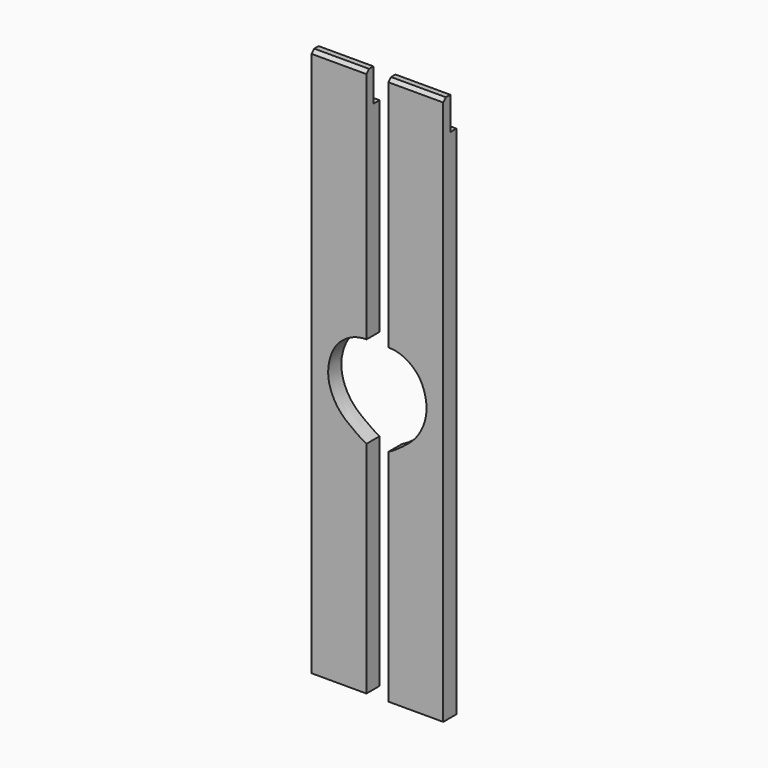
from build123d import *

# Parameters (mm, degrees)
F0_W     = 63.5
F0_H     = 635
F1_DEPTH = 19.05
F2_DEPTH = 19.05
F4_DEPTH = 25.4
F5_W     = 8.89
F5_H     = 38.1
F6_DEPTH = 203.2


# Not quite as in the source:
# - ends of sketch curves that miss each other by under 0.0002 mm in the source are joined
# - the dataset's text gives a spline's control points without its knots; the knots are read off the source's solid


with BuildPart() as f1:
    # F0 (on Front) → F1 (new body)
    with BuildSketch(Plane.XZ):
        with Locations((31.75, 317.5)):
            Rectangle(F0_W, F0_H)
    extrude(amount=F1_DEPTH)

    # F0 (on Front) → F2 (join)
    with BuildSketch(Plane.XZ):
        with Locations((31.75, 317.5)):
            Rectangle(F0_W, F0_H)
    extrude(amount=F2_DEPTH)


with BuildPart() as f2:
    # F0 (on Front) → F2, piece 2 (new body)
    with BuildSketch(Plane.XZ):
        with Locations((120.65, 317.5)):
            Rectangle(F0_W, F0_H)
    extrude(amount=F2_DEPTH)


with BuildPart() as f4_tool:
    # F3 (on Front) → F4 (new body)
    with BuildSketch(Plane.XZ):
        with BuildLine():
            add(Edge.make_bspline(
                [(76.100897188, 249.9055047823), (75.926185189, 249.9503102981), (75.0072900635, 250.1900406969), (73.2686411586, 250.6826857781), (70.8066541331, 251.4744223929), (68.2535936156, 252.4016337409), (66.0855662311, 253.2919660254), (64.3444467026, 254.0808435025), (62.6141081034, 254.9200047281), (60.530623259, 256.0298058039), (58.1240131579, 257.4465535403), (55.796019872, 258.9289142825), (53.5234926315, 260.4628622816), (51.6580388559, 261.7732381383), (50.1690572917, 262.8373998229), (49.0559378965, 263.6386485181), (47.9204267705, 264.459940904), (46.3757335395, 265.5883530434), (44.4005510811, 267.0614970435), (41.9904856802, 268.940615508), (39.5721301398, 270.9437516515), (37.1771637761, 273.0857076613), (35.2273267058, 275.0014654048), (33.7139364208, 276.6200965999), (32.6031412309, 277.8843862966), (31.5392969514, 279.1785289773), (30.1869925643, 280.9326379146), (28.6162502842, 283.1744606608), (26.9167867496, 285.9192166814), (25.3965198658, 288.697331361), (24.0503105367, 291.4878274589), (22.8732786897, 294.2731728334), (21.8629980956, 297.0286748974), (21.0083636149, 299.7731949442), (20.0799064427, 303.4278925622), (19.3201051185, 307.9921101901), (19.0525714688, 313.46912822), (19.3407698255, 318.0082202574), (19.8503150972, 321.6100699757), (20.3651164621, 324.2955196511), (20.8994087113, 326.5198480427), (21.3857760258, 328.2896704175), (21.9199810431, 330.0777026424), (22.6836120267, 332.3350954426), (23.7765594955, 335.0624054196), (25.0695252606, 337.7860696689), (26.5870492336, 340.482876144), (28.0551387249, 342.6818667185), (29.3671419532, 344.4023295399), (30.7492710306, 346.0639842696), (32.5901917449, 348.0257211027), (35.741037592, 350.9238010664), (39.1454385563, 353.4591937744), (42.7161593673, 355.6127823059), (45.4584424247, 357.0273277396), (48.2564247079, 358.2324558767), (51.1102551, 359.2200466799), (54.0138871108, 359.9816388995), (56.9592002347, 360.5106156141), (59.4398513134, 360.7540031429), (61.4342021839, 360.8300374212), (63.4344324402, 360.8265137523), (65.8869615803, 360.6817979446), (68.7271248443, 360.3158428641), (70.9786334936, 359.8645110662), (72.7038693594, 359.4132156878), (73.9618405888, 359.0249055159), (74.9862735439, 358.6517484591), (75.6947865713, 358.3571550213), (75.9996347623, 358.2212228776), (76.1008674062, 358.1750149305)],
                knots=[0.0119144147, 0.0119144147, 0.0119144147, 0.0119144147, 0.015625, 0.03125, 0.046875, 0.0625, 0.078125, 0.0859375, 0.09375, 0.109375, 0.125, 0.140625, 0.15625, 0.171875, 0.1796875, 0.1875, 0.1953125, 0.203125, 0.21875, 0.234375, 0.25, 0.265625, 0.28125, 0.2890625, 0.296875, 0.3046875, 0.3125, 0.328125, 0.34375, 0.359375, 0.375, 0.390625, 0.40625, 0.421875, 0.4375, 0.46875, 0.5, 0.53125, 0.546875, 0.5625, 0.578125, 0.5859375, 0.59375, 0.609375, 0.625, 0.640625, 0.65625, 0.671875, 0.6796875, 0.6875, 0.703125, 0.71875, 0.75, 0.765625, 0.78125, 0.796875, 0.8125, 0.828125, 0.84375, 0.859375, 0.8671875, 0.875, 0.890625, 0.90625, 0.921875, 0.9296875, 0.9375, 0.9453125, 0.94921875, 0.9511701686, 0.9511701686, 0.9511701686, 0.9511701686], degree=3))
            add(Edge.make_bspline(
                [(76.100897188, 249.9055047823), (76.2756168386, 249.9503111688), (77.1945168439, 250.1900430656), (78.9331699313, 250.682690976), (81.3951543845, 251.4744307141), (83.9482096728, 252.4016452369), (86.116231215, 253.2919796709), (87.8573457702, 254.0808583153), (89.5876785997, 254.9200197664), (91.6711580774, 256.029820577), (94.0777640591, 257.4465674509), (96.405755399, 258.9289272147), (98.6782824462, 260.4628744396), (100.5437371698, 261.7732500288), (102.0327198813, 262.837411785), (103.145840351, 263.6386607264), (104.2813528676, 264.4599537749), (105.8260473996, 265.5883666646), (107.8012309574, 267.0615116848), (110.2112968302, 268.9406314175), (112.6296521558, 270.9437688896), (115.0246177189, 273.0857262522), (116.9744537113, 275.0014851029), (118.4878429498, 276.6201171365), (119.5986372357, 277.8844074231), (120.6624802917, 279.1785501954), (122.0147832858, 280.9326593221), (123.5855239506, 283.1744821164), (125.2849858024, 285.9192380456), (126.8052511868, 288.6973524974), (128.1514591642, 291.487848283), (129.3284897486, 294.2731932749), (130.3387691649, 297.0286950062), (131.1934024624, 299.773214912), (132.1218579887, 303.4279122656), (132.881657234, 307.9921294882), (133.149188649, 313.4691466183), (132.8609888351, 318.0082378668), (132.3514425295, 321.6100870656), (131.8366404312, 324.2955364489), (131.3023476205, 326.519864578), (130.8159798099, 328.2896870107), (130.2817741986, 330.0777194315), (129.5181424112, 332.335112362), (128.4251938616, 335.0624223728), (127.1322269153, 337.7860864558), (125.614701652, 340.4828925104), (124.1466109752, 342.6818824907), (122.8346067266, 344.4023445867), (121.4524770025, 346.0639980719), (119.6115556172, 348.0257332111), (116.4607092605, 350.9238100822), (113.0563086511, 353.4591996745), (109.4855891414, 355.6127862016), (106.7433080737, 357.0273308598), (103.9453270996, 358.2324600721), (101.0914966428, 359.220053263), (98.1878630338, 359.981648241), (95.2425465495, 360.5106269364), (92.7618912668, 360.7540143035), (90.767536362, 360.830046655), (88.7673018665, 360.8265195246), (86.3147732106, 360.6817972563), (83.4746173865, 360.3158348795), (81.2231208145, 359.8645006778), (79.4978993004, 359.4132086375), (78.2399418313, 359.0249048351), (77.2155240176, 358.6517580268), (76.5070027285, 358.3571668032), (76.2021400516, 358.2212307008), (76.1008674062, 358.1750149305)],
                knots=[0.0119143513, 0.0119143513, 0.0119143513, 0.0119143513, 0.015625, 0.03125, 0.046875, 0.0625, 0.078125, 0.0859375, 0.09375, 0.109375, 0.125, 0.140625, 0.15625, 0.171875, 0.1796875, 0.1875, 0.1953125, 0.203125, 0.21875, 0.234375, 0.25, 0.265625, 0.28125, 0.2890625, 0.296875, 0.3046875, 0.3125, 0.328125, 0.34375, 0.359375, 0.375, 0.390625, 0.40625, 0.421875, 0.4375, 0.46875, 0.5, 0.53125, 0.546875, 0.5625, 0.578125, 0.5859375, 0.59375, 0.609375, 0.625, 0.640625, 0.65625, 0.671875, 0.6796875, 0.6875, 0.703125, 0.71875, 0.75, 0.765625, 0.78125, 0.796875, 0.8125, 0.828125, 0.84375, 0.859375, 0.8671875, 0.875, 0.890625, 0.90625, 0.921875, 0.9296875, 0.9375, 0.9453125, 0.94921875, 0.9511705713, 0.9511705713, 0.9511705713, 0.9511705713], degree=3))
        make_face()
        with BuildLine():
            add(Edge.make_bspline(
                [(76.1008975875, 257.8056084785), (78.8384725301, 258.603465596), (86.9111078068, 261.4830017438), (98.5683426497, 269.6292487284), (114.611152191, 281.5212568651), (123.4921764827, 298.1418802401), (126.1504124582, 312.0828373038), (124.2309410858, 325.807586611), (118.2536925199, 340.2351730196), (104.4132884729, 350.8872381857), (90.7850560754, 354.1803431207), (79.1363194034, 351.8571206075), (76.9024601615, 349.743447754), (76.1008841428, 348.9886770249)],
                knots=[0.0265026492, 0.0265026492, 0.0265026492, 0.0265026492, 0.0875905171, 0.1858081447, 0.2951543718, 0.4004723033, 0.4916695348, 0.5816823509, 0.6775492616, 0.7781334208, 0.8705307121, 0.9523354115, 0.9998266821, 0.9998266821, 0.9998266821, 0.9998266821], degree=3))
            add(Edge.make_bspline(
                [(76.1008975875, 257.8056084785), (73.3633126459, 258.6034660297), (65.290644766, 261.4829960162), (53.6334221611, 269.6292504895), (37.5906072531, 281.5212564236), (28.7095843098, 298.1418802436), (26.0513476326, 312.082836876), (27.9708197396, 325.8075871319), (33.9480672966, 340.2351702939), (47.7884749561, 350.8872480286), (61.4166908867, 354.1803183251), (73.0654809705, 351.8571479661), (75.2992625877, 349.7434038281), (76.1008841428, 348.9886770248)],
                knots=[0.0265027098, 0.0265027098, 0.0265027098, 0.0265027098, 0.0875906622, 0.1858082813, 0.2951544964, 0.4004724176, 0.4916696401, 0.5816824478, 0.6775493491, 0.7781335021, 0.8705307722, 0.9523354596, 0.999826872, 0.999826872, 0.999826872, 0.999826872], degree=3))
        make_face(mode=Mode.SUBTRACT)
        with BuildLine():
            add(Edge.make_bspline(
                [(76.1008975875, 257.8056084785), (73.3633126459, 258.6034660297), (65.290644766, 261.4829960162), (53.6334221611, 269.6292504895), (37.5906072531, 281.5212564236), (28.7095843098, 298.1418802436), (26.0513476326, 312.082836876), (27.9708197396, 325.8075871319), (33.9480672966, 340.2351702939), (47.7884749561, 350.8872480286), (61.4166908867, 354.1803183251), (73.0654809705, 351.8571479661), (75.2992625877, 349.7434038281), (76.1008841428, 348.9886770248)],
                knots=[0.0265027098, 0.0265027098, 0.0265027098, 0.0265027098, 0.0875906622, 0.1858082813, 0.2951544964, 0.4004724176, 0.4916696401, 0.5816824478, 0.6775493491, 0.7781335021, 0.8705307722, 0.9523354596, 0.999826872, 0.999826872, 0.999826872, 0.999826872], degree=3))
            add(Edge.make_bspline(
                [(76.1008975875, 257.8056084785), (78.8384725301, 258.603465596), (86.9111078068, 261.4830017438), (98.5683426497, 269.6292487284), (114.611152191, 281.5212568651), (123.4921764827, 298.1418802401), (126.1504124582, 312.0828373038), (124.2309410858, 325.807586611), (118.2536925199, 340.2351730196), (104.4132884729, 350.8872381857), (90.7850560754, 354.1803431207), (79.1363194034, 351.8571206075), (76.9024601615, 349.743447754), (76.1008841428, 348.9886770249)],
                knots=[0.0265026492, 0.0265026492, 0.0265026492, 0.0265026492, 0.0875905171, 0.1858081447, 0.2951543718, 0.4004723033, 0.4916695348, 0.5816823509, 0.6775492616, 0.7781334208, 0.8705307121, 0.9523354115, 0.9998266821, 0.9998266821, 0.9998266821, 0.9998266821], degree=3))
        make_face()
    extrude(amount=F4_DEPTH)


with BuildPart() as f1_1:
    add(f1.part)

    # F4: cut by f4_tool
    add(f4_tool.part, mode=Mode.SUBTRACT)


with BuildPart() as f2_1:
    add(f2.part)

    # F4: cut by f4_tool
    add(f4_tool.part, mode=Mode.SUBTRACT)


with BuildPart() as f6_tool:
    # F5 (on face) → F6 (new body)
    with BuildSketch(Plane.YZ.offset(152.4)):
        Polygon((-19.05, 631.19), (-15.24, 635), (-19.05, 635), align=None)
        with Locations((-4.445, 615.95)):
            Rectangle(F5_W, F5_H)
    extrude(amount=-F6_DEPTH)


with BuildPart() as f1_2:
    add(f1_1.part)

    # F6: cut by f6_tool
    add(f6_tool.part, mode=Mode.SUBTRACT)


with BuildPart() as f2_2:
    add(f2_1.part)

    # F6: cut by f6_tool
    add(f6_tool.part, mode=Mode.SUBTRACT)


solid = Compound([f1_2.part, f2_2.part])
